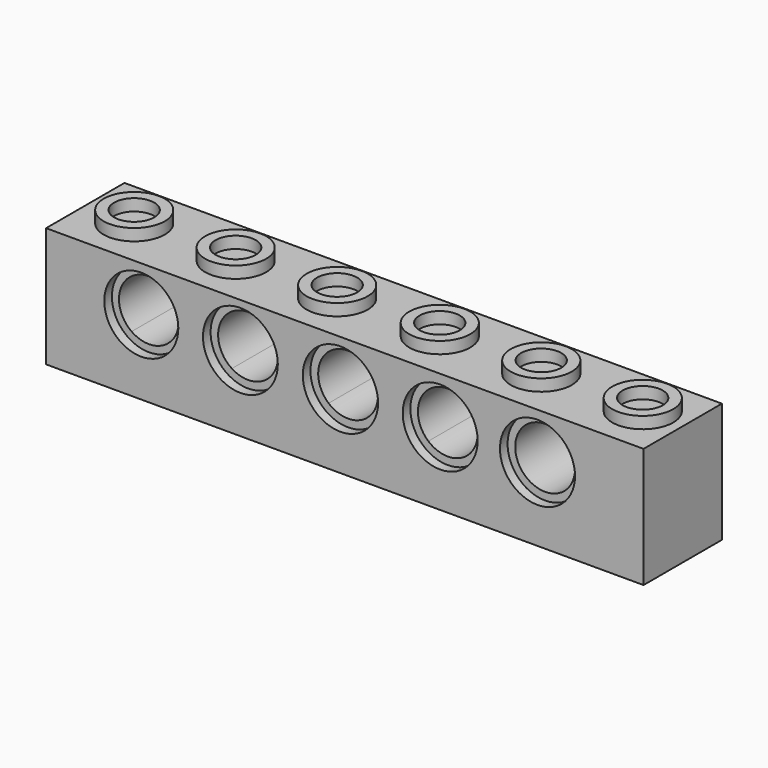
from build123d import *

# Parameters (mm, degrees)
F0_W      = 47.7012
F0_H      = 9.5758
F1_DEPTH  = 7.8232
F2_R      = 2.3876
F3_DEPTH  = 9.53232
F2_R_2    = 3.0048968535
F2_R_3    = 2.9922132855
F2_R_4    = 2.9972531663
F4_DEPTH  = 0.762
F5_R      = 2.9885913722
F5_R_2    = 3.0048968535
F5_R_3    = 2.9922132855
F5_R_4    = 2.9972531663
F5_R_5    = 2.9570387739
F6_DEPTH  = 25.4
F7_R      = 3.0048968535
F7_R_2    = 2.3876
F7_R_3    = 2.9922132855
F7_R_4    = 2.9972531663
F7_R_5    = 2.9885913722
F7_R_6    = 2.9570387739
F8_DEPTH  = 0.762
F9_R      = 2.4384
F9_R_2    = 1.6002
F10_DEPTH = 0.9398
F11_W     = 45.9232
F11_H     = 6.0452
F12_DEPTH = 2.794


with BuildPart() as f1:
    # F0 (on Front) → F1 (new body)
    with BuildSketch(Plane.XZ):
        with Locations((-0.3360249102, 0.7659190055)):
            Rectangle(F0_W, F0_H)
    extrude(amount=F1_DEPTH)

    # F2 (on Front) → F3 (cut)
    with BuildSketch(Plane.XZ):
        with Locations((15.0480590754, 1.8556544835)):
            Circle(F2_R)
        with BuildLine():
            Line((5.7234941433, 0), (8.8326681668, 3.624302958))
            ThreePointArc((8.8326681668, 3.624302958), (5.4659296761, 3.3667384908), (5.7234941433, 0))
        make_face()
        with BuildLine():
            ThreePointArc((5.7234941433, 0), (8.275302748, -0.3572223603), (9.6656811551, 1.812151479))
            ThreePointArc((9.6656811551, 1.812151479), (9.4474549944, 2.8093730719), (8.8326681668, 3.624302958))
            Line((8.8326681668, 3.624302958), (5.7234941433, 0))
        make_face()
        with BuildLine():
            Line((-2.2399391754, 0.0756290061), (0.8692348481, 3.6999319641))
            ThreePointArc((0.8692348481, 3.6999319641), (-2.4975036427, 3.4423674968), (-2.2399391754, 0.0756290061))
        make_face()
        with BuildLine():
            ThreePointArc((-2.2399391754, 0.0756290061), (0.3118694292, -0.2815933542), (1.7022478363, 1.8877804851))
            ThreePointArc((1.7022478363, 1.8877804851), (1.4840216756, 2.885002078), (0.8692348481, 3.6999319641))
            Line((0.8692348481, 3.6999319641), (-2.2399391754, 0.0756290061))
        make_face()
        with BuildLine():
            Line((-9.9647576041, 0), (-7.3799977582, 4.0151651995))
            ThreePointArc((-7.3799977582, 4.0151651995), (-10.6799602808, 3.2999625227), (-9.9647576041, 0))
        make_face()
        with BuildLine():
            ThreePointArc((-9.9647576041, 0), (-7.5289295065, -0.0884040491), (-6.2847776811, 2.0075825997))
            ThreePointArc((-6.2847776811, 2.0075825997), (-6.5763910323, 3.1510307743), (-7.3799977582, 4.0151651995))
            Line((-7.3799977582, 4.0151651995), (-9.9647576041, 0))
        make_face()
        with BuildLine():
            Line((-17.9671654597, 0), (-15.2041278281, 3.8946319578))
            ThreePointArc((-15.2041278281, 3.8946319578), (-18.5329626228, 3.3288347947), (-17.9671654597, 0))
        make_face()
        with BuildLine():
            ThreePointArc((-17.9671654597, 0), (-15.4897179429, -0.1739039631), (-14.1980466439, 1.9473159789))
            ThreePointArc((-14.1980466439, 1.9473159789), (-14.4644267019, 3.0432446799), (-15.2041278281, 3.8946319578))
            Line((-15.2041278281, 3.8946319578), (-17.9671654597, 0))
        make_face()
    extrude(amount=F3_DEPTH, mode=Mode.SUBTRACT)

    # F2 (on Front) → F4 (cut)
    with BuildSketch(Plane.XZ):
        with BuildLine():
            ThreePointArc((-16.5209776811, 4.9036475293), (-16.5856466439, 4.9043547528), (-16.6503156067, 4.9036475293))
            Line((-16.6503156067, 4.9036475293), (-16.5209776811, 4.9036475293))
        make_face()
        with BuildLine():
            ThreePointArc((-5.6837863089, 2.0075825997), (-6.8384723861, 4.3673431298), (-9.41027084, 4.9036475293))
            ThreePointArc((-9.41027084, 4.9036475293), (-10.5062829761, -0.3521779303), (-5.6837863089, 2.0075825997))
        make_face()
        with BuildLine():
            ThreePointArc((-7.3799977582, 4.0151651995), (-6.5763910323, 3.1510307743), (-6.2847776811, 2.0075825997))
            ThreePointArc((-6.2847776811, 2.0075825997), (-7.5289295065, -0.0884040491), (-9.9647576041, 0))
            ThreePointArc((-9.9647576041, 0), (-10.6799602808, 3.2999625227), (-7.3799977582, 4.0151651995))
        make_face(mode=Mode.SUBTRACT)
        with BuildLine():
            Line((-16.5209776811, 4.9036475293), (-16.6503156067, 4.9036475293))
            ThreePointArc((-16.6503156067, 4.9036475293), (-18.5630084962, 4.1459788488), (-19.5185854293, 2.3240763694))
            ThreePointArc((-19.5185854293, 2.3240763694), (-18.8162584098, 0.0060665204), (-16.6174061088, -1.0095522371))
            ThreePointArc((-16.6174061088, -1.0095522371), (-14.5059634539, -0.1548248679), (-13.6286078699, 1.9473159789))
            ThreePointArc((-13.6286078699, 1.9473159789), (-14.4719642007, 4.0152678256), (-16.5209776811, 4.9036475293))
        make_face()
        with BuildLine():
            ThreePointArc((-15.2041278281, 3.8946319578), (-14.4644267019, 3.0432446799), (-14.1980466439, 1.9473159789))
            ThreePointArc((-14.1980466439, 1.9473159789), (-15.4897179429, -0.1739039631), (-17.9671654597, 0))
            ThreePointArc((-17.9671654597, 0), (-18.5329626228, 3.3288347947), (-15.2041278281, 3.8946319578))
        make_face(mode=Mode.SUBTRACT)
        with Locations((-0.6853521637, 1.8877804851)):
            Circle(F2_R_2)
        with BuildLine():
            ThreePointArc((0.8692348481, 3.6999319641), (1.4840216756, 2.885002078), (1.7022478363, 1.8877804851))
            ThreePointArc((1.7022478363, 1.8877804851), (0.3118694292, -0.2815933542), (-2.2399391754, 0.0756290061))
            ThreePointArc((-2.2399391754, 0.0756290061), (-2.4975036427, 3.4423674968), (0.8692348481, 3.6999319641))
        make_face(mode=Mode.SUBTRACT)
        with Locations((7.2780811551, 1.812151479)):
            Circle(F2_R_3)
        with BuildLine():
            ThreePointArc((8.8326681668, 3.624302958), (9.4474549944, 2.8093730719), (9.6656811551, 1.812151479))
            ThreePointArc((9.6656811551, 1.812151479), (8.275302748, -0.3572223603), (5.7234941433, 0))
            ThreePointArc((5.7234941433, 0), (5.4659296761, 3.3667384908), (8.8326681668, 3.624302958))
        make_face(mode=Mode.SUBTRACT)
        with Locations((15.0480590754, 1.8556544835)):
            Circle(F2_R_4)
        with Locations((15.0480590754, 1.8556544835)):
            Circle(F2_R, mode=Mode.SUBTRACT)
    extrude(amount=F4_DEPTH, mode=Mode.SUBTRACT)

    # F5 (on Front) → F6 (cut)
    with BuildSketch(Plane.XZ):
        with Locations((-8.6723776811, 2.0075825997)):
            Circle(F5_R)
        with Locations((-0.6853521637, 1.8877804851)):
            Circle(F5_R_2)
        with Locations((7.2780811551, 1.812151479)):
            Circle(F5_R_3)
        with Locations((15.0480590754, 1.8556544835)):
            Circle(F5_R_4)
        with Locations((-16.5856466439, 1.9473159789)):
            Circle(F5_R_5)
    extrude(amount=-F6_DEPTH, mode=Mode.SUBTRACT)

    # F7 (on face) → F8 (cut)
    with BuildSketch(Plane.XZ.offset(7.8232)):
        with Locations((-0.6853521637, 1.8877804851)):
            Circle(F7_R)
        with Locations((-0.6853521637, 1.8877804851)):
            Circle(F7_R_2, mode=Mode.SUBTRACT)
        with Locations((7.2780811551, 1.812151479)):
            Circle(F7_R_3)
        with Locations((7.2780811551, 1.812151479)):
            Circle(F7_R_2, mode=Mode.SUBTRACT)
        with Locations((15.0480590754, 1.8556544835)):
            Circle(F7_R_4)
        with Locations((15.0480590754, 1.8556544835)):
            Circle(F7_R_2, mode=Mode.SUBTRACT)
        with Locations((-8.6723776811, 2.0075825997)):
            Circle(F7_R_5)
        with Locations((-8.6723776811, 2.0075825997)):
            Circle(F7_R_2, mode=Mode.SUBTRACT)
        with Locations((-16.5856466439, 1.9473159789)):
            Circle(F7_R_6)
        with Locations((-16.5856466439, 1.9473159789)):
            Circle(F7_R_2, mode=Mode.SUBTRACT)
    extrude(amount=-F8_DEPTH, mode=Mode.SUBTRACT)

    # F9 (on face) → F10 (join)
    with BuildSketch(Plane.XY.offset(5.5538190055)):
        with Locations((-20.3004249102, -3.8862)):
            Circle(F9_R)
        with Locations((-20.3004249102, -3.8862)):
            Circle(F9_R_2, mode=Mode.SUBTRACT)
        with Locations((-12.1978249102, -3.8862)):
            Circle(F9_R)
        with Locations((-12.1978249102, -3.8862)):
            Circle(F9_R_2, mode=Mode.SUBTRACT)
        with Locations((-4.0952249102, -3.8862)):
            Circle(F9_R)
        with Locations((-4.0952249102, -3.8862)):
            Circle(F9_R_2, mode=Mode.SUBTRACT)
        with Locations((4.0952249102, -3.8862)):
            Circle(F9_R)
        with Locations((4.0952249102, -3.8862)):
            Circle(F9_R_2, mode=Mode.SUBTRACT)
        with Locations((12.1978249102, -3.8862)):
            Circle(F9_R)
        with Locations((12.1978249102, -3.8862)):
            Circle(F9_R_2, mode=Mode.SUBTRACT)
        with Locations((20.3004249102, -3.8862)):
            Circle(F9_R)
        with Locations((20.3004249102, -3.8862)):
            Circle(F9_R_2, mode=Mode.SUBTRACT)
    extrude(amount=F10_DEPTH)

    # F11 (on face) → F12 (cut)
    with BuildSketch(Plane(origin=(0, 0, -4.0219809945), x_dir=(1, 0, 0), z_dir=(0, 0, -1))):
        with Locations((-0.3360249102, 3.9116)):
            Rectangle(F11_W, F11_H)
    extrude(amount=-F12_DEPTH, mode=Mode.SUBTRACT)


solid = f1.part
